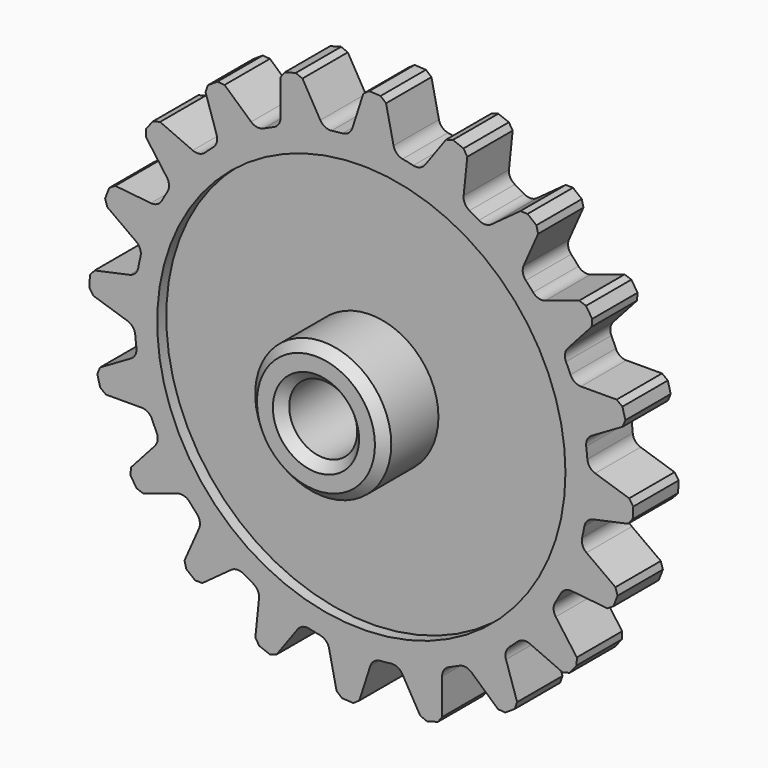
from build123d import *

# Parameters (mm, degrees)
F0_R            = 100
F1_DEPTH        = 25
F3_DEPTH        = 25
F3_COPIES_COUNT = 20
F4_SIZE         = 2
F5_R            = 5
F6_R            = 90
F7_DEPTH        = 5
F8_R            = 30
F9_DEPTH        = 30
F10_R           = 15
F11_DEPTH       = 50.001
F12_SIZE        = 4


# Not quite as in the source:
# - a pattern or mirror of a feature is missing from the dataset's text; its kind, count and spacing are read off the source's solid


with BuildPart() as f1:
    # F0 (on Front) → F1 (new body)
    with BuildSketch(Plane.XZ):
        Circle(F0_R)
    extrude(amount=F1_DEPTH)

    # F2 (on face) → F3 (join)
    with BuildSketch(Plane.XZ.offset(25)):
        Polygon((-61.7759852264, 102.8772455371), (-69.3126066074, 97.9579632561), (-62.7351563306, 77.8736165859), (-46.0375728595, 88.7724162407), align=None)
        with BuildLine():
            Line((-61.7759852264, 102.8772455371), (-69.3126066074, 97.9579632561))
            Line((-69.3126066074, 97.9579632561), (-62.7351563306, 77.8736165859))
            ThreePointArc((-62.7351563306, 77.8736165859), (-54.6586920109, 83.7402375663), (-46.0375728595, 88.7724162407))
            Line((-46.0375728595, 88.7724162407), (-61.7759852264, 102.8772455371))
        make_face()
    f3 = extrude(amount=-F3_DEPTH)

    # F3_copies: F3 ×20 about axis
    f3_copies_axis = Axis((0, 0, 0), (0, 1, 0))
    for i in range(1, F3_COPIES_COUNT):
        add(f3.rotate(f3_copies_axis, i * 360 / F3_COPIES_COUNT))

    # F4
    f4_edges = [f1.edges().sort_by_distance(p)[0] for p in [
        (-61.775985, -12.5, 102.877246),
        (-69.312607, -12.5, 97.957963),
        (-90.543271, -12.5, 78.752245),
        (78.752245, -12.5, 90.543271),
        (97.957963, -12.5, 69.312607),
        (102.877246, -12.5, 61.775985),
        (114.582333, -12.5, 35.649531),
        (116.931904, -12.5, 26.961636),
        (119.990585, -12.5, -1.503169),
        (119.540453, -12.5, -10.491906),
        (113.653323, -12.5, -38.508729),
        (110.44755, -12.5, -46.918427),
        (96.190882, -12.5, -71.744786),
        (90.543271, -12.5, -78.752245),
        (69.312607, -12.5, -97.957963),
        (61.775985, -12.5, -102.877246),
        (35.649531, -12.5, -114.582333),
        (26.961636, -12.5, -116.931904),
        (-1.503169, -12.5, -119.990585),
        (-10.491906, -12.5, -119.540453),
        (-38.508729, -12.5, -113.653323),
        (-46.918427, -12.5, -110.44755),
        (-71.744786, -12.5, -96.190882),
        (-78.752245, -12.5, -90.543271),
        (-97.957963, -12.5, -69.312607),
        (-102.877246, -12.5, -61.775985),
        (-114.582333, -12.5, -35.649531),
        (-116.931904, -12.5, -26.961636),
        (-119.990585, -12.5, 1.503169),
        (-119.540453, -12.5, 10.491906),
        (-113.653323, -12.5, 38.508729),
        (-110.44755, -12.5, 46.918427),
        (-35.649531, -12.5, 114.582333),
        (-26.961636, -12.5, 116.931904),
        (1.503169, -12.5, 119.990585),
        (10.491906, -12.5, 119.540453),
        (38.508729, -12.5, 113.653323),
        (46.918427, -12.5, 110.44755),
        (71.744786, -12.5, 96.190882),
        (-96.190882, -12.5, 71.744786),
    ]]
    chamfer(f4_edges, length=F4_SIZE)

    # F5
    f5_edges = [f1.edges().sort_by_distance(p)[0] for p in [
        (-46.037573, -12.5, 88.772416),
        (-62.735156, -12.5, 77.873617),
        (70.201193, -12.5, 71.216519),
        (77.873617, -12.5, 62.735156),
        (54.675981, -12.5, 83.72895),
        (44.758187, -12.5, 89.424296),
        (88.772416, -12.5, 46.037573),
        (93.44844, -12.5, 35.600408),
        (26.12628, -12.5, 96.526771),
        (14.933938, -12.5, 98.8786),
        (98.653977, -12.5, 16.352148),
        (99.875879, -12.5, 4.980844),
        (-4.980844, -12.5, 99.875879),
        (-16.352148, -12.5, 98.653977),
        (98.8786, -12.5, -14.933938),
        (96.526771, -12.5, -26.12628),
        (-35.600408, -12.5, 93.44844),
        (89.424296, -12.5, -44.758187),
        (83.72895, -12.5, -54.675981),
        (-71.216519, -12.5, 70.201193),
        (71.216519, -12.5, -70.201193),
        (62.735156, -12.5, -77.873617),
        (-83.72895, -12.5, 54.675981),
        (-89.424296, -12.5, 44.758187),
        (46.037573, -12.5, -88.772416),
        (35.600408, -12.5, -93.44844),
        (-96.526771, -12.5, 26.12628),
        (-98.8786, -12.5, 14.933938),
        (16.352148, -12.5, -98.653977),
        (4.980844, -12.5, -99.875879),
        (-99.875879, -12.5, -4.980844),
        (-98.653977, -12.5, -16.352148),
        (-14.933938, -12.5, -98.8786),
        (-26.12628, -12.5, -96.526771),
        (-93.44844, -12.5, -35.600408),
        (-88.772416, -12.5, -46.037573),
        (-44.758187, -12.5, -89.424296),
        (-54.675981, -12.5, -83.72895),
        (-77.873617, -12.5, -62.735156),
        (-70.201193, -12.5, -71.216519),
    ]]
    fillet(f5_edges, radius=F5_R)

    # F6 (on face) → F7 (cut)
    with BuildSketch(Plane.XZ.offset(25)):
        Circle(F6_R)
    extrude(amount=-F7_DEPTH, mode=Mode.SUBTRACT)

    # F8 (on face) → F9 (join)
    with BuildSketch(Plane.XZ.offset(20)):
        Circle(F8_R)
    extrude(amount=F9_DEPTH)

    # F10 (on face) → F11 (cut, through all)
    with BuildSketch(Plane.XZ.offset(50)):
        Circle(F10_R)
    extrude(amount=-F11_DEPTH, mode=Mode.SUBTRACT)

    # F12
    f12_edges = [f1.edges().sort_by_distance(p)[0] for p in [
        (-15, -50, 0),
        (-30, -50, 0),
    ]]
    chamfer(f12_edges, length=F12_SIZE)


solid = f1.part
